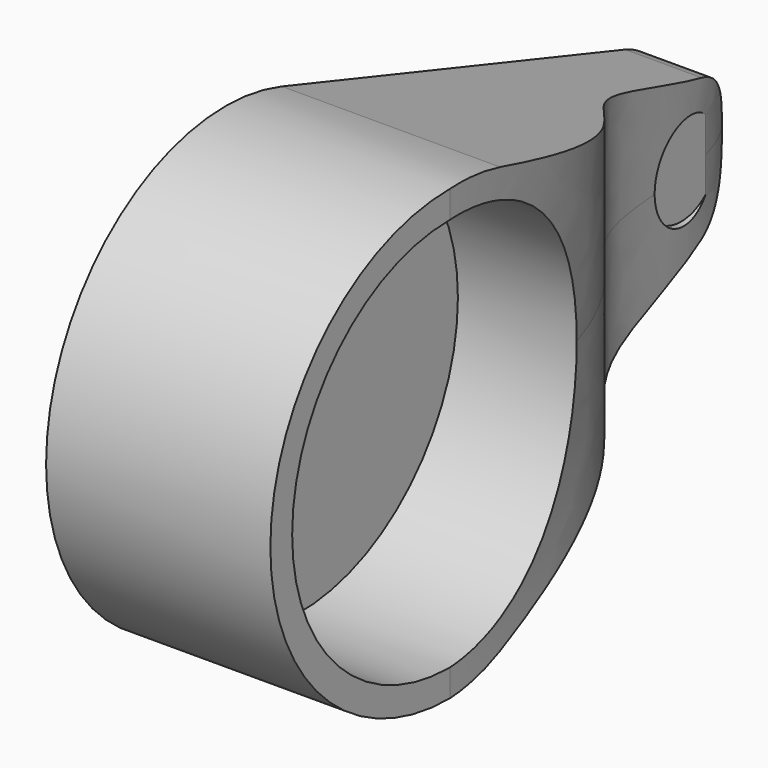
from build123d import *

# Parameters (mm, degrees)
F1_DEPTH = 76.2
F2_R     = 66.9441745007
F2_R_2   = 15.875
F3_DEPTH = 50.8
F5_DEPTH = 137.16


# Not quite as in the source:
# - a feature names something its author has since deleted; it is built from what else it names


with BuildPart() as f1:
    # F0 (on Right) → F1 (new body)
    with BuildSketch(Plane.YZ):
        with BuildLine():
            Line((169.7282094477, 24.1148148653), (23.9315970236, 72.344444596))
            ThreePointArc((23.9315970236, 72.344444596), (-76.2, 0), (23.9315970236, -72.344444596))
            Line((23.9315970236, -72.344444596), (169.7282094477, -24.1148148653))
            ThreePointArc((169.7282094477, -24.1148148653), (187.1510104398, 0), (169.7282094477, 24.1148148653))
        make_face()
    extrude(amount=F1_DEPTH)

    # F2 (on face) → F3 (cut)
    with BuildSketch(Plane.YZ.offset(76.2)):
        Circle(F2_R)
        with Locations((161.7510104398, 0)):
            Circle(F2_R_2)
    extrude(amount=-F3_DEPTH, mode=Mode.SUBTRACT)

    # F4 (on Top) → F5 (cut, symmetric)
    with BuildSketch(Plane.XY):
        with BuildLine():
            add(Edge.make_bspline(
                [(76.2, 0), (69.7670128122, 106.6320095463), (15.5509841332, 89.3209706266), (33.872663393, 196.783595894), (-4.8366077244, 199.8663842678)],
                knots=[0, 0, 0, 0, 0.5611625531, 1, 1, 1, 1], degree=3))
            Line((76.2, 0), (76.2, 199.8663842678))
            Line((76.2, 199.8663842678), (-4.8366077244, 199.8663842678))
        make_face()
    extrude(amount=F5_DEPTH, both=True, mode=Mode.SUBTRACT)


solid = f1.part
